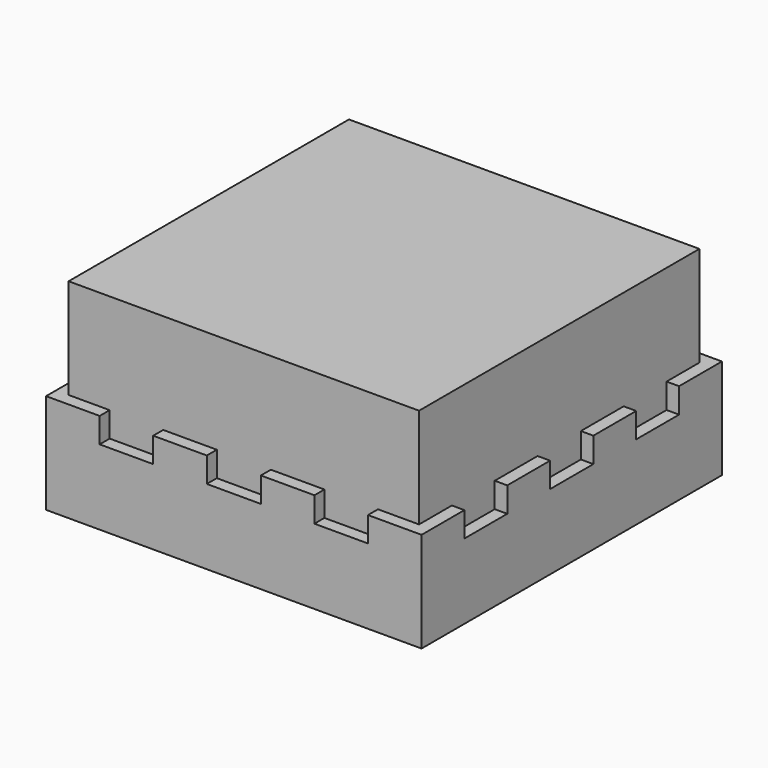
from build123d import *

# Parameters (mm, degrees)
F0_W      = 140
F0_H      = 140
F1_DEPTH  = 40
F4_DEPTH  = 145
F5_DEPTH  = 145
F6_DEPTH  = 5
F7_DEPTH  = 5
F2_W      = 5
F2_H      = 40
F8_DEPTH  = 5
F9_DEPTH  = 5
F10_W     = 10
F10_H     = 10
F11_DEPTH = 3.5
F10_W_2   = 20
F10_H_2   = 20
F12_DEPTH = 5


with BuildPart() as f1:
    # F0 (on Top) → F1 (new body, symmetric)
    with BuildSketch(Plane.XY):
        Rectangle(F0_W, F0_H)
    extrude(amount=F1_DEPTH, both=True)

    # F3 (on face) → F4 (join)
    with BuildSketch(Plane(origin=(-70, 0, 0), x_dir=(0, -1, 0), z_dir=(-1, 0, 0))):
        Polygon((-70, -40), (70, -40), (70, 0), (53.6, 0), (53.6, -10), (32.2, -10), (32.2, 0), (10.8, 0), (10.8, -10), (-10.8, -10), (-10.8, 0), (-32.2, 0), (-32.2, -10), (-53.6, -10), (-53.6, 0), (-70, 0), align=None)
    extrude(amount=-F4_DEPTH)

    # F2 (on face) → F5 (join)
    with BuildSketch(Plane(origin=(0, 70, 0), x_dir=(-1, 0, 0), z_dir=(0, 1, 0))):
        Polygon((-70, -40), (70, -40), (70, 0), (53.6, 0), (53.6, -10), (32.2, -10), (32.2, 0), (10.8, 0), (10.8, -10), (-10.8, -10), (-10.8, 0), (-32.2, 0), (-32.2, -10), (-53.6, -10), (-53.6, 0), (-70, 0), align=None)
    extrude(amount=-F5_DEPTH)

    # F2 (on face) → F6 (join)
    with BuildSketch(Plane(origin=(0, 70, 0), x_dir=(-1, 0, 0), z_dir=(0, 1, 0))):
        Polygon((-70, -40), (70, -40), (70, 0), (53.6, 0), (53.6, -10), (32.2, -10), (32.2, 0), (10.8, 0), (10.8, -10), (-10.8, -10), (-10.8, 0), (-32.2, 0), (-32.2, -10), (-53.6, -10), (-53.6, 0), (-70, 0), align=None)
    extrude(amount=F6_DEPTH)

    # F3 (on face) → F7 (join)
    with BuildSketch(Plane(origin=(-70, 0, 0), x_dir=(0, -1, 0), z_dir=(-1, 0, 0))):
        Polygon((-70, -40), (70, -40), (70, 0), (53.6, 0), (53.6, -10), (32.2, -10), (32.2, 0), (10.8, 0), (10.8, -10), (-10.8, -10), (-10.8, 0), (-32.2, 0), (-32.2, -10), (-53.6, -10), (-53.6, 0), (-70, 0), align=None)
    extrude(amount=F7_DEPTH)

    # F2 (on face) → F8 (join, through all)
    with BuildSketch(Plane(origin=(0, 70, 0), x_dir=(-1, 0, 0), z_dir=(0, 1, 0))):
        with Locations((-72.5, -20)):
            Rectangle(F2_W, F2_H)
        with Locations((72.5, -20)):
            Rectangle(F2_W, F2_H)
    extrude(amount=F8_DEPTH)

    # F9 (add, through all): faces of the model
    f9_faces = [f1.faces().sort_by_distance(p)[0] for p in [
        (72.5, -70, -20),
        (-72.5, -70, -20),
    ]]
    extrude(f9_faces, amount=F9_DEPTH)

    # F10 (on face) → F11 (join)
    with BuildSketch(Plane(origin=(0, 0, -40), x_dir=(1, 0, 0), z_dir=(0, 0, -1))):
        with Locations((-55, 5)):
            Rectangle(F10_W, F10_H)
        with Locations((-35, -15)):
            Rectangle(F10_W, F10_H)
        with Locations((-45, -55)):
            Rectangle(F10_W, F10_H)
        with Locations((25, 15)):
            Rectangle(F10_W, F10_H)
        with Locations((15, 35)):
            Rectangle(F10_W, F10_H)
        with Locations((45, 55)):
            Rectangle(F10_W, F10_H)
    extrude(amount=F11_DEPTH)

    # F10 (on face) → F12 (join)
    with BuildSketch(Plane(origin=(0, 0, -40), x_dir=(1, 0, 0), z_dir=(0, 0, -1))):
        with Locations((40, -10)):
            Rectangle(F10_W_2, F10_H_2)
        Rectangle(F10_W_2, F10_H_2)
        with Locations((-40, 30)):
            Rectangle(F10_W_2, F10_H_2)
        with Locations((10, -40)):
            Rectangle(F10_W_2, F10_H_2)
    extrude(amount=F12_DEPTH)


solid = f1.part
